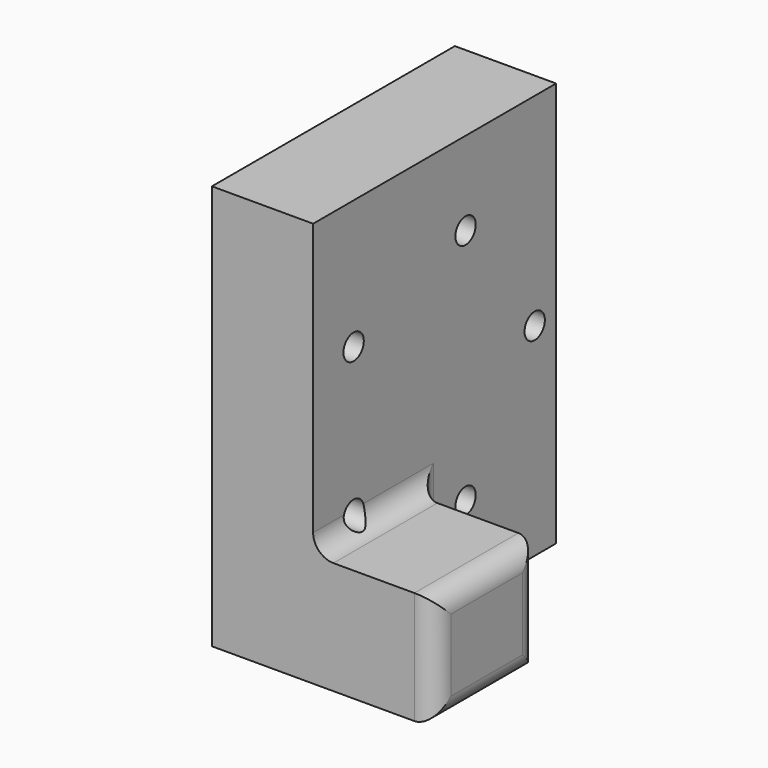
from build123d import *

# Parameters (mm, degrees)
F0_W         = 76.2
F0_H         = 101.6
F1_DEPTH     = 25.4
F3_D         = 6.3754
F4_W         = 32.6189571008
F4_H         = 28.2830937386
F5_DEPTH     = 30.48
F6_T1_DEPTH  = 28.2830937386
F6_T6_DEPTH  = 32.6189571008
F6_S7_R      = 3.1877
F6_T8_DEPTH  = 18
F6_T13_DEPTH = 40.9830937386
F6_T17_DEPTH = 45.3189571008
F6_T20_DEPTH = 53.6830937386
F6_T22_DEPTH = 58.0189571008


# Not quite as in the source:
# - a fillet or chamfer that OpenCascade refuses, or shapes differently, is made with other operations: its cross-section is extruded or revolved along the edge and cut away or added


with BuildPart() as f1:
    # F0 (on Right) → F1 (new body)
    with BuildSketch(Plane.YZ):
        Rectangle(F0_W, F0_H)
    extrude(amount=F1_DEPTH)

    # F3 (through all)
    with Locations(Plane(origin=(0, 0, 0), x_dir=(0, -1, 0), z_dir=(-1, 0, 0))):
        with Locations((-31.3961266285, 0), (-9.7019366858, 29.8594908165), (25.4, 18.4541802113), (25.4, -18.4541802113), (-9.7019366858, -29.8594908165)):
            Hole(F3_D / 2)

    # F4 (on face) → F5 (join)
    with BuildSketch(Plane.YZ.offset(25.4)):
        with Locations((-21.7905214496, -36.6584531307)):
            Rectangle(F4_W, F4_H)
    extrude(amount=F5_DEPTH)

    # F6: fillet of radius 5.08 on 6 edges, made by hand

    # F6_s2 → F6_t1 (join)
    with BuildSketch(Plane.XY.offset(-50.8)):
        with BuildLine():
            ThreePointArc((25.4, -0.4010428992), (26.8878975516, -3.9931453476), (30.48, -5.4810428992))
            Line((30.48, -5.4810428992), (25.4, -5.4810428992))
            Line((25.4, -5.4810428992), (25.4, -0.4010428992))
        make_face()
    extrude(amount=F6_T1_DEPTH)


with BuildPart() as f6_tool4:
    # F6_s5 → F6_t6 (new body)
    with BuildSketch(Plane.XZ.offset(5.4810428992)):
        with BuildLine():
            ThreePointArc((25.4, -17.4369062614), (26.8878975516, -21.0290087099), (30.48, -22.5169062614))
            Line((30.48, -22.5169062614), (25.4, -22.5169062614))
            Line((25.4, -22.5169062614), (25.4, -17.4369062614))
        make_face()
    extrude(amount=F6_T6_DEPTH)

    # F6_s7 → F6_t8 (cut, symmetric)
    with BuildSketch(Plane.YZ.offset(27.9)):
        with Locations((-25.4, -18.4541802113)):
            Circle(F6_S7_R)
    extrude(amount=F6_T8_DEPTH, both=True, mode=Mode.SUBTRACT)


with BuildPart() as f1_1:
    add(f1.part)

    # F6_t3: union F6_tool4
    add(f6_tool4.part)


with BuildPart() as f6_tool11:
    # F6_s12 → F6_t13 (new body)
    with BuildSketch(Plane.XY.offset(-50.8)):
        with BuildLine():
            ThreePointArc((25.4, -0.4010428992), (26.8878975516, -3.9931453476), (30.48, -5.4810428992))
            Line((30.48, -5.4810428992), (25.4, -5.4810428992))
            Line((25.4, -5.4810428992), (25.4, -0.4010428992))
        make_face()
    extrude(amount=F6_T13_DEPTH)

    split(bisect_by=Plane.XY.offset(-22.5169062614), keep=Keep.TOP)


with BuildPart() as f6_tool15:
    # F6_s16 → F6_t17 (new body)
    with BuildSketch(Plane.XZ.offset(-7.2189571008)):
        with BuildLine():
            ThreePointArc((25.4, -17.4369062614), (26.8878975516, -21.0290087099), (30.48, -22.5169062614))
            Line((30.48, -22.5169062614), (25.4, -22.5169062614))
            Line((25.4, -22.5169062614), (25.4, -17.4369062614))
        make_face()
    extrude(amount=F6_T17_DEPTH)

    split(bisect_by=Plane.XZ.offset(5.4810428992), keep=Keep.BOTTOM)


with BuildPart() as f6_tool11_1:
    add(f6_tool11.part)

    # F6_t19: intersect F6_tool15
    add(f6_tool15.part, mode=Mode.INTERSECT)


with BuildPart() as f1_2:
    add(f1_1.part)

    # F6_t9: union F6_tool11
    add(f6_tool11_1.part)

    # F6_s21 → F6_t20 (cut)
    with BuildSketch(Plane.XY.offset(-63.5)):
        with BuildLine():
            ThreePointArc((50.8, -5.4810428992), (54.3921024484, -6.9689404508), (55.88, -10.5610428992))
            Line((55.88, -10.5610428992), (55.88, -5.4810428992))
            Line((55.88, -5.4810428992), (50.8, -5.4810428992))
        make_face()
        with BuildLine():
            ThreePointArc((55.88, -33.02), (54.3921024484, -36.6121024484), (50.8, -38.1))
            Line((50.8, -38.1), (55.88, -38.1))
            Line((55.88, -38.1), (55.88, -33.02))
        make_face()
    extrude(amount=F6_T20_DEPTH, mode=Mode.SUBTRACT)

    # F6_s23 → F6_t22 (cut)
    with BuildSketch(Plane.XZ.offset(-7.2189571008)):
        with BuildLine():
            ThreePointArc((55.88, -45.72), (54.3921024484, -49.3121024484), (50.8, -50.8))
            Line((50.8, -50.8), (55.88, -50.8))
            Line((55.88, -50.8), (55.88, -45.72))
        make_face()
        with BuildLine():
            ThreePointArc((55.88, -27.5969062614), (54.3921024484, -24.004803813), (50.8, -22.5169062614))
            Line((50.8, -22.5169062614), (55.88, -22.5169062614))
            Line((55.88, -22.5169062614), (55.88, -27.5969062614))
        make_face()
    extrude(amount=F6_T22_DEPTH, mode=Mode.SUBTRACT)


solid = f1_2.part
